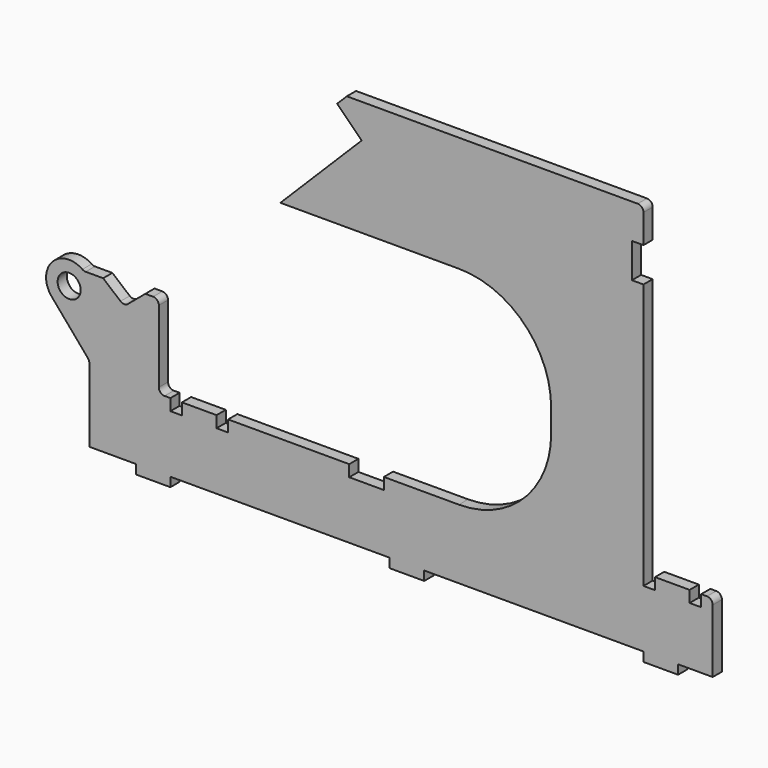
from build123d import *

# Parameters (mm, degrees)
F0_R     = 6.35
F0_W     = 19.05
F0_H     = 5.08
F1_DEPTH = 6.35
F2_R     = 3.175
F3_R     = 5.08
F4_R     = 3.175
F5_R     = 3.175


# Not quite as in the source:
# - ends of sketch curves that miss each other by under 0.0002 mm in the source are joined


with BuildPart() as f1:
    # F0 (on Front) → F1 (new body)
    with BuildSketch(Plane.XZ):
        with BuildLine():
            Line((-72.7094654823, -50.272475262), (-83.3648741359, -50.272475262))
            ThreePointArc((-83.3648741359, -50.272475262), (-100.4842470659, -51.222143603), (-101.056400417, -68.3582903151))
            Line((-101.056400417, -68.3582903151), (-80.147210941, -92.8018072064))
            Line((-80.147210941, -92.8018072064), (-80.147210941, -134.409975262))
            Line((-80.147210941, -134.409975262), (-54.747210941, -134.409975262))
            Line((-54.747210941, -134.409975262), (-35.697210941, -134.409975262))
            Line((-35.697210941, -134.409975262), (84.952789059, -134.409975262))
            Line((84.952789059, -134.409975262), (104.002789059, -134.409975262))
            Line((104.002789059, -134.409975262), (224.652789059, -134.409975262))
            Line((224.652789059, -134.409975262), (243.702789059, -134.409975262))
            Line((243.702789059, -134.409975262), (262.752789059, -134.409975262))
            Line((262.752789059, -134.409975262), (262.752789059, -96.309975262))
            Line((262.752789059, -96.309975262), (256.402789059, -96.309975262))
            Line((256.402789059, -96.309975262), (256.402789059, -102.659975262))
            Line((256.402789059, -102.659975262), (250.052789059, -102.659975262))
            Line((250.052789059, -102.659975262), (250.052789059, -96.309975262))
            Line((250.052789059, -96.309975262), (231.002789059, -96.309975262))
            Line((231.002789059, -96.309975262), (231.002789059, -102.659975262))
            Line((231.002789059, -102.659975262), (224.652789059, -102.659975262))
            Line((224.652789059, -102.659975262), (224.652789059, 43.390024738))
            Line((224.652789059, 43.390024738), (218.302789059, 43.390024738))
            Line((218.302789059, 43.390024738), (218.302789059, 62.440024738))
            Line((218.302789059, 62.440024738), (224.652789059, 62.440024738))
            Line((224.652789059, 62.440024738), (224.652789059, 81.490024738))
            Line((224.652789059, 81.490024738), (61.4126609984, 81.490024738))
            Line((61.4126609984, 81.490024738), (56.0792184251, 76.1565821646))
            Line((56.0792184251, 76.1565821646), (69.5496026067, 62.686197983))
            Line((69.5496026067, 62.686197983), (24.8534293616, 17.990024738))
            Line((24.8534293616, 17.990024738), (123.052789059, 17.990024738))
            ThreePointArc((123.052789059, 17.990024738), (158.9738135432, 3.1110492223), (173.852789059, -32.809975262))
            Line((173.852789059, -32.809975262), (173.852789059, -45.509975262))
            ThreePointArc((173.852789059, -45.509975262), (158.9738135432, -81.4309997463), (123.052789059, -96.309975262))
            Line((123.052789059, -96.309975262), (81.777789059, -96.309975262))
            Line((81.777789059, -96.309975262), (81.777789059, -102.659975262))
            Line((81.777789059, -102.659975262), (62.727789059, -102.659975262))
            Line((62.727789059, -102.659975262), (62.727789059, -96.309975262))
            Line((62.727789059, -96.309975262), (-3.947210941, -96.309975262))
            Line((-3.947210941, -96.309975262), (-3.947210941, -102.659975262))
            Line((-3.947210941, -102.659975262), (-10.297210941, -102.659975262))
            Line((-10.297210941, -102.659975262), (-10.297210941, -96.309975262))
            Line((-10.297210941, -96.309975262), (-29.347210941, -96.309975262))
            Line((-29.347210941, -96.309975262), (-29.347210941, -102.659975262))
            Line((-29.347210941, -102.659975262), (-35.697210941, -102.659975262))
            Line((-35.697210941, -102.659975262), (-35.697210941, -96.309975262))
            Line((-35.697210941, -96.309975262), (-42.047210941, -96.309975262))
            Line((-42.047210941, -96.309975262), (-42.047210941, -50.272475262))
            Line((-42.047210941, -50.272475262), (-49.4849563998, -50.272475262))
            Line((-49.4849563998, -50.272475262), (-61.097210941, -60.0163137647))
            Line((-61.097210941, -60.0163137647), (-72.7094654823, -50.272475262))
        make_face()
        with Locations((-91.4055753496, -60.1028935639)):
            Circle(F0_R, mode=Mode.SUBTRACT)
        with Locations((-45.222210941, -136.949975262)):
            Rectangle(F0_W, F0_H)
        with Locations((94.477789059, -136.949975262)):
            Rectangle(F0_W, F0_H)
        with Locations((234.177789059, -136.949975262)):
            Rectangle(F0_W, F0_H)
    extrude(amount=-F1_DEPTH)

    # F2
    f2_edges = [f1.edges().sort_by_distance(p)[0] for p in [
        (224.652789, 3.175, 81.490025),
        (-42.047211, 3.175, -96.309975),
    ]]
    fillet(f2_edges, radius=F2_R)

    # F3
    f3_edges = [f1.edges().sort_by_distance(p)[0] for p in [
        (-80.147211, 3.175, -92.801807),
    ]]
    fillet(f3_edges, radius=F3_R)

    # F4
    f4_edges = [f1.edges().sort_by_distance(p)[0] for p in [
        (-42.047211, 3.175, -50.272475),
    ]]
    fillet(f4_edges, radius=F4_R)

    # F5
    f5_edges = [f1.edges().sort_by_distance(p)[0] for p in [
        (-61.097211, 3.175, -60.016314),
        (-83.364874, 3.175, -50.272475),
        (262.752789, 3.175, -96.309975),
    ]]
    fillet(f5_edges, radius=F5_R)


solid = f1.part
